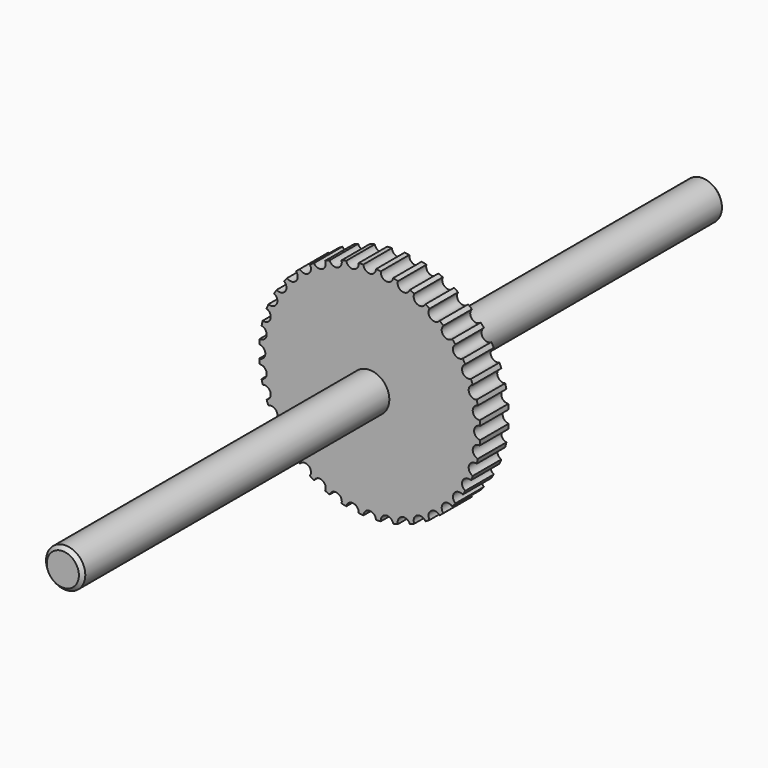
from build123d import *

# Parameters (mm, degrees)
F0_R            = 7.874
F0_R_2          = 6.985
F0_R_3          = 1.397
F1_DEPTH        = 1.27
F2_DEPTH        = 28.575
F4_DEPTH        = 25.4
F4_COPIES_COUNT = 40
F5_SIZE         = 0.254


# Not quite as in the source:
# - a pattern or mirror of a feature is missing from the dataset's text; its kind, count and spacing are read off the source's solid


with BuildPart() as f1:
    # F0 (on Front) → F1 (new body, symmetric)
    with BuildSketch(Plane.XZ):
        Circle(F0_R)
        Circle(F0_R_2, mode=Mode.SUBTRACT)
        Circle(F0_R_2)
        Circle(F0_R_3, mode=Mode.SUBTRACT)
    extrude(amount=F1_DEPTH, both=True)

    # F0 (on Front) → F2 (join, symmetric)
    with BuildSketch(Plane.XZ):
        Circle(F0_R_3)
    extrude(amount=F2_DEPTH, both=True)

    # F3 (on face) → F4 (cut)
    with BuildSketch(Plane.XZ.offset(1.27)):
        with BuildLine():
            ThreePointArc((0.444322899, 7.861453629), (0, 7.874), (-0.444322899, 7.861453629))
            ThreePointArc((-0.444322899, 7.861453629), (0, 7.4295), (0.444322899, 7.861453629))
        make_face()
    f4 = extrude(amount=-F4_DEPTH, mode=Mode.SUBTRACT)

    # F4_copies: F4 ×40 about axis
    f4_copies_axis = Axis((0, 0, 0), (0, 1, 0))
    for i in range(1, F4_COPIES_COUNT):
        add(f4.rotate(f4_copies_axis, i * 360 / F4_COPIES_COUNT), mode=Mode.SUBTRACT)

    # F5
    f5_edges = [f1.edges().sort_by_distance(p)[0] for p in [
        (-1.397, -28.575, 0),
        (-1.397, 28.575, 0),
    ]]
    chamfer(f5_edges, length=F5_SIZE)


solid = f1.part
